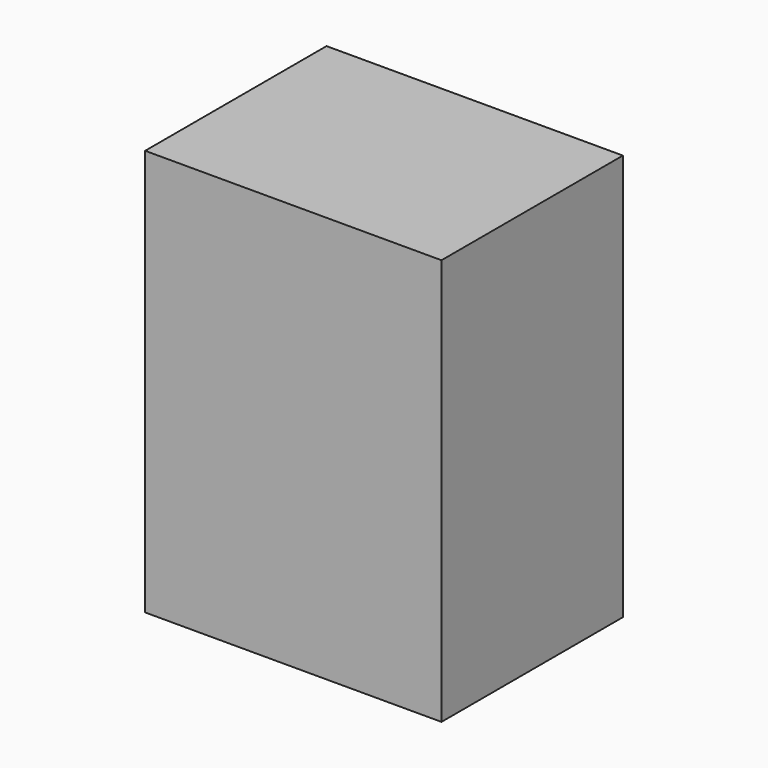
from build123d import *

# Parameters (mm, degrees)
F0_W     = 630
F0_H     = 482
F1_DEPTH = 864


# Not quite as in the source:
# - the program builds the solid bodies; features that only make, move or delete a surface that nothing else refers to are left out


with BuildPart() as f1:
    # F0 (on Top) → F1 (new body)
    with BuildSketch(Plane.XY):
        with Locations((15.069953084, -49.194766596)):
            Rectangle(F0_W, F0_H)
    extrude(amount=F1_DEPTH)


solid = f1.part
